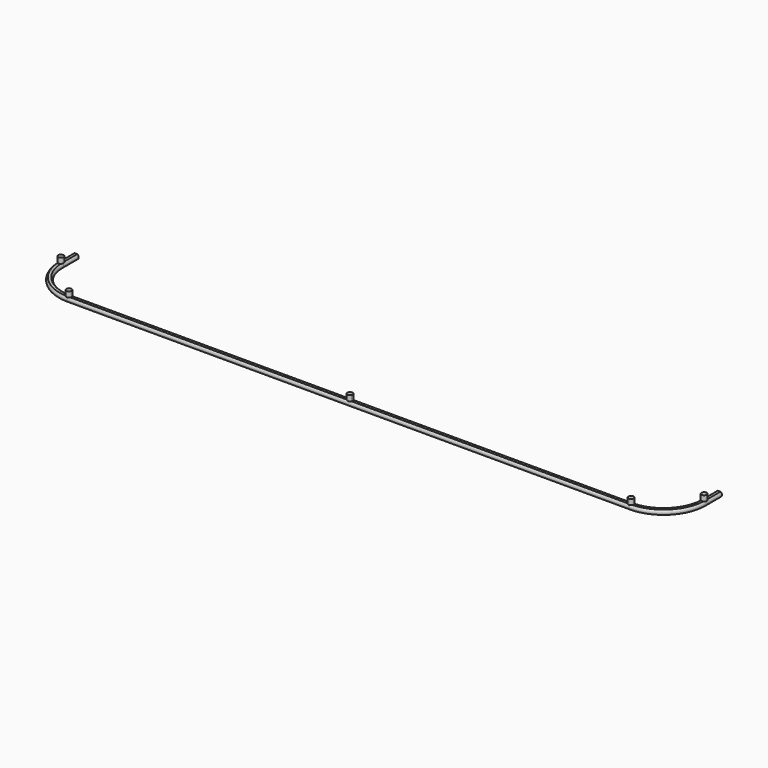
from build123d import *

# Parameters (mm, degrees)
F3_R     = 10
F4_DEPTH = 20
F6_DEPTH = 20


with BuildPart() as f2:
    # F2: sweep along a path in F1
    with BuildLine(Plane.XY) as f2_path:
        Line((0, 0), (0, -70))
        ThreePointArc((0, -70), (43.933982822, -176.066017178), (150, -220))
        Line((150, -220), (2230, -220))
        ThreePointArc((2230, -220), (2336.066017178, -176.066017178), (2380, -70))
        Line((2380, -70), (2380, 0))
    # F0 (on Front) → F2 (sweep)
    with BuildSketch(Plane.XZ):
        with BuildLine():
            Line((0, 8.6602540378), (-5, 8.6602540378))
            ThreePointArc((-5, 8.6602540378), (-10, 0), (-5, -8.6602540378))
            Line((-5, -8.6602540378), (5, -8.6602540378))
            ThreePointArc((5, -8.6602540378), (10, 0), (5, 8.6602540378))
            Line((5, 8.6602540378), (0, 8.6602540378))
        make_face()
    sweep(path=f2_path.line)

    # F3 (on face) → F4 (join)
    with BuildSketch(Plane.XY.offset(8.6602540378)):
        with Locations((0, -70)):
            Circle(F3_R)
        with Locations((150, -220)):
            Circle(F3_R)
        with Locations((2380, -70)):
            Circle(F3_R)
        with Locations((2230, -220)):
            Circle(F3_R)
    extrude(amount=F4_DEPTH)

    # F5 (on face) → F6 (join)
    with BuildSketch(Plane.XY.offset(8.6602540378)):
        with BuildLine():
            Line((1198.6602540378, -215), (1190, -215))
            Line((1190, -215), (1190, -220))
            Line((1190, -220), (1190, -225))
            Line((1190, -225), (1198.6602540378, -225))
            ThreePointArc((1198.6602540378, -225), (1199.6592582629, -222.588190451), (1200, -220))
            ThreePointArc((1200, -220), (1199.6592582629, -217.411809549), (1198.6602540378, -215))
        make_face()
        with BuildLine():
            Line((1181.3397459622, -215), (1190, -215))
            Line((1190, -215), (1198.6602540378, -215))
            ThreePointArc((1198.6602540378, -215), (1190, -210), (1181.3397459622, -215))
        make_face()
        with BuildLine():
            Line((1190, -220), (1190, -215))
            Line((1190, -215), (1181.3397459622, -215))
            ThreePointArc((1181.3397459622, -215), (1180.3407417371, -217.411809549), (1180, -220))
            Line((1180, -220), (1190, -220))
        make_face()
        with BuildLine():
            Line((1190, -225), (1190, -220))
            Line((1190, -220), (1180, -220))
            ThreePointArc((1180, -220), (1180.3407417371, -222.588190451), (1181.3397459622, -225))
            Line((1181.3397459622, -225), (1190, -225))
        make_face()
        with BuildLine():
            Line((1198.6602540378, -225), (1190, -225))
            Line((1190, -225), (1181.3397459622, -225))
            ThreePointArc((1181.3397459622, -225), (1190, -230), (1198.6602540378, -225))
        make_face()
    extrude(amount=F6_DEPTH)


solid = f2.part
